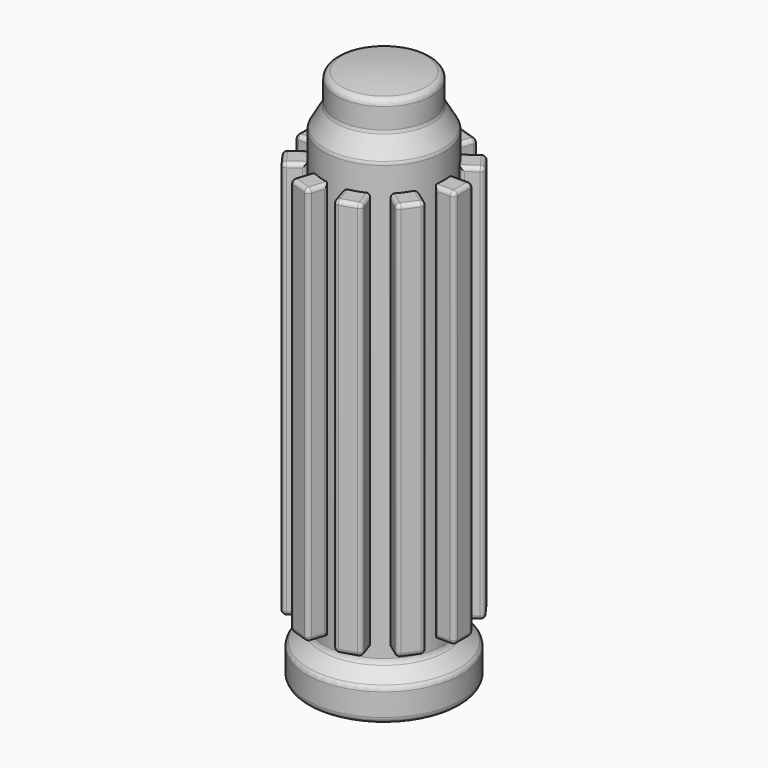
from build123d import *

# Parameters (mm, degrees)
F2_R     = 1.6
F4_W     = 6
F4_H     = 100
F6_R     = 1
F7_COUNT = 10


with BuildPart() as f1:
    # F0 (on Front) → F1 (revolve)
    with BuildSketch(Plane.XZ):
        with BuildLine():
            Line((10.75, 125), (10.75, 0))
            Line((10.75, 0), (19.325, 0))
            Line((19.325, 0), (19.325, 8))
            Line((19.325, 8), (15, 11.6291059048))
            Line((15, 11.6291059048), (15, 121.6291059048))
            Line((15, 121.6291059048), (11.8991128484, 127))
            Line((11.8991128484, 127), (11.8991128484, 133.9508111483))
            ThreePointArc((11.8991128484, 133.9508111483), (5.9726393626, 134.7371949452), (0, 135))
            Line((0, 135), (0, 125))
            Line((0, 125), (10.75, 125))
        make_face()
    revolve(axis=Axis((0, 0, 66.9849514961), (0, 0, 1)))

    # F2
    f2_edges = [f1.edges().sort_by_distance(p)[0] for p in [
        (-15, 0, 11.629106),
        (-19.325, 0, 8),
        (-19.325, 0, 0),
        (-15, 0, 121.629106),
        (-11.899113, 0, 127),
        (-11.899113, 0, 133.950811),
    ]]
    fillet(f2_edges, radius=F2_R)


with BuildPart() as f5:
    # F4 (on offset) → F5 (new body, up to the next surface of F1)
    with BuildSketch(Plane.YZ.offset(20)):
        with Locations((4.657e-07, 65)):
            Rectangle(F4_W, F4_H)
    extrude(until=Until.NEXT, target=f1.part, dir=(-1, 0, 0))

    # F6
    f6_edges = [f5.edges().sort_by_distance(p)[0] for p in [
        (20, 0, 115),
        (20, -3, 65),
        (14.696939, -3, 65),
        (20, 3, 65),
        (14.696938, 3, 65),
        (17.348469, 3, 15),
        (20, 0, 15),
        (17.348469, 3, 115),
        (17.348469, -3, 115),
        (17.348469, -3, 15),
    ]]
    fillet(f6_edges, radius=F6_R)


with BuildPart() as f7_1:
    # F7: instance of F5
    add(f5.part.rotate(Axis((0, 0, 66.9849514961), (0, 0, 1)), 1 * 360 / F7_COUNT))


with BuildPart() as f7_2:
    # F7: instance of F5
    add(f5.part.rotate(Axis((0, 0, 66.9849514961), (0, 0, 1)), 2 * 360 / F7_COUNT))


with BuildPart() as f7_3:
    # F7: instance of F5
    add(f5.part.rotate(Axis((0, 0, 66.9849514961), (0, 0, 1)), 3 * 360 / F7_COUNT))


with BuildPart() as f7_4:
    # F7: instance of F5
    add(f5.part.rotate(Axis((0, 0, 66.9849514961), (0, 0, 1)), 4 * 360 / F7_COUNT))


with BuildPart() as f7_5:
    # F7: instance of F5
    add(f5.part.rotate(Axis((0, 0, 66.9849514961), (0, 0, 1)), 5 * 360 / F7_COUNT))


with BuildPart() as f7_6:
    # F7: instance of F5
    add(f5.part.rotate(Axis((0, 0, 66.9849514961), (0, 0, 1)), 6 * 360 / F7_COUNT))


with BuildPart() as f7_7:
    # F7: instance of F5
    add(f5.part.rotate(Axis((0, 0, 66.9849514961), (0, 0, 1)), 7 * 360 / F7_COUNT))


with BuildPart() as f7_8:
    # F7: instance of F5
    add(f5.part.rotate(Axis((0, 0, 66.9849514961), (0, 0, 1)), 8 * 360 / F7_COUNT))


with BuildPart() as f7_9:
    # F7: instance of F5
    add(f5.part.rotate(Axis((0, 0, 66.9849514961), (0, 0, 1)), 9 * 360 / F7_COUNT))


solid = Compound([f1.part, f5.part, f7_1.part, f7_2.part, f7_3.part, f7_4.part, f7_5.part, f7_6.part, f7_7.part, f7_8.part, f7_9.part])
